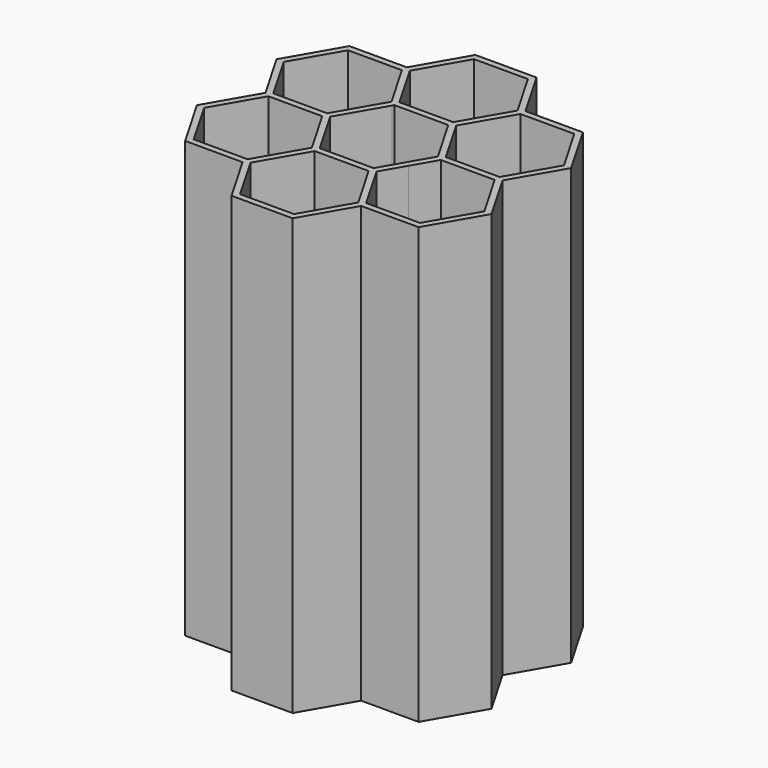
from build123d import *

# Parameters (mm, degrees)
F1_DEPTH = 140


# Not quite as in the source:
# - ends of sketch curves that miss each other by under 0.0002 mm in the source are joined


with BuildPart() as f1:
    # F0 (on Top) → F1 (new body)
    with BuildSketch(Plane.XY):
        Polygon((9.8149545762, -17), (19.0525588833, -1), (37.5277626519, -1), (47.3427172281, 16), (38.1051129211, 32), (47.3427172281, 48), (37.5277626519, 65), (19.0525576719, 65), (9.8149545762, 81), (-9.8149545762, 81), (-19.0525576719, 65.0000020981), (-37.5277626519, 65), (-47.3427172281, 48), (-38.1051129211, 32), (-47.3427172281, 16), (-37.5277626519, -1), (-19.0525588833, -1), (-9.8149545762, -17), align=None)
        Polygon((-10.3923048454, 16), (-19.0525576719, 1.0000020981), (-36.3730621135, 1), (-45.0333161514, 16), (-36.3730621135, 31), (-19.0525540378, 31), align=None, mode=Mode.SUBTRACT)
        Polygon((-17.3205080757, 0), (-8.6602540378, 15), (8.6602540378, 15), (17.3205080757, 0), (8.6602540378, -15), (-8.6602540378, -15), align=None, mode=Mode.SUBTRACT)
        Polygon((8.6602540378, 17), (-8.6602540378, 17), (-17.3205080757, 32), (-8.9903810568, 46.4282032303), (-8.6602540378, 47), (8.6602540378, 47), (16.9903849907, 32.5717899559), (17.3205080757, 32), align=None, mode=Mode.SUBTRACT)
        Polygon((19.0525576719, 1.0000020981), (10.3923048454, 16), (14.7224318643, 23.5), (19.0525540378, 31), (36.3730621135, 31), (45.0333161514, 16), (36.3730621135, 1), align=None, mode=Mode.SUBTRACT)
        Polygon((-10.3923048454, 48), (-19.0525576719, 33.0000020981), (-36.3730621135, 33), (-45.0333161514, 48), (-36.3730621135, 63), (-19.0525540378, 63), align=None, mode=Mode.SUBTRACT)
        Polygon((19.0525576719, 33.0000020981), (10.3923048454, 48), (19.0525576719, 62.9999979019), (36.3730621135, 63), (45.0333161514, 48), (36.3730621135, 33), align=None, mode=Mode.SUBTRACT)
        Polygon((8.6602540378, 49), (-8.6602540378, 49), (-17.3205080757, 64), (-8.6602540378, 79), (8.6602540378, 79), (17.3205080757, 64), align=None, mode=Mode.SUBTRACT)
    extrude(amount=F1_DEPTH)


solid = f1.part
